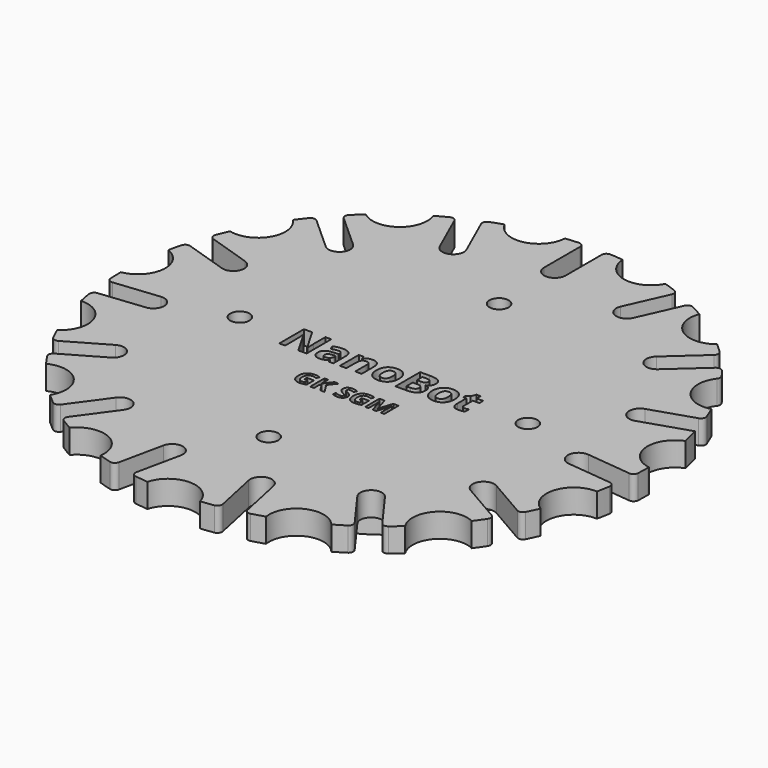
from build123d import *

# Parameters (mm, degrees)
F1_DEPTH       = 6
F2_DEPTH       = 6
F2_DEPTH_BACK  = 13
F3_DEPTH       = 2
F4_R           = 2
F5_DEPTH       = 10
F6_DEPTH       = 3
F7_TEXT_SIZE   = 8.9862398203
F7_TEXT_SIZE_2 = 5.2074857608
F8_DEPTH       = 3
F9_R           = 1
F10_DEPTH      = 1


# Not quite as in the source:
# - Text() gives the source's letters only with a copy of the font that has no kerning and outlines rounded to 1/6400 em; it was checked with that copy


with BuildPart() as f1:
    # F0 (on Top) → F1 (new body)
    with BuildSketch(Plane.XY):
        with BuildLine():
            ThreePointArc((54.8881035117, -3.5065785158), (54.9720187602, -1.7541816975), (55, 0))
            ThreePointArc((55, 0), (54.9998451105, 0.1305289846), (54.9993804431, 0.261057234))
            ThreePointArc((54.9993804431, 0.261057234), (50.2561749386, 5.2821368343), (53.8517888732, 11.1796616747))
            ThreePointArc((53.8517888732, 11.1796616747), (53.4370798147, 13.0183908712), (52.9596080906, 14.8418297689))
            Line((52.9596080906, 14.8418297689), (43.0553454731, 11.6237397678))
            ThreePointArc((43.0553454731, 11.6237397678), (40.2201800741, 13.0683286921), (41.6647689984, 15.9034940911))
            Line((41.6647689984, 15.9034940911), (51.5690316159, 19.1215840922))
            ThreePointArc((51.5690316159, 19.1215840922), (50.8835238625, 20.8774279865), (50.1382526339, 22.608751023))
            ThreePointArc((50.1382526339, 22.608751023), (43.7628617294, 25.2665), (44.6488790507, 32.1166249708))
            ThreePointArc((44.6488790507, 32.1166249708), (43.5221449332, 33.6277103058), (42.3442933924, 35.0992993819))
            Line((42.3442933924, 35.0992993819), (34.6052143911, 28.1310013499))
            ThreePointArc((34.6052143911, 28.1310013499), (31.4275946694, 28.2975333429), (31.5941266625, 31.4751530645))
            Line((31.5941266625, 31.4751530645), (39.3332056638, 38.4434510965))
            ThreePointArc((39.3332056638, 38.4434510965), (37.9927971182, 39.768673188), (36.6077654526, 41.047186366))
            ThreePointArc((36.6077654526, 41.047186366), (29.7025521541, 40.8820557767), (27.725772418, 47.5003320391))
            ThreePointArc((27.725772418, 47.5003320391), (26.0818358065, 48.4224931304), (24.4072656808, 49.2877812646))
            Line((24.4072656808, 49.2877812646), (20.1715273623, 39.7741572365))
            ThreePointArc((20.1715273623, 39.7741572365), (18.9223779691, 38.5887587238), (17.2008926357, 38.6338374037))
            Line((17.2008926357, 38.6338374037), (8.7448378261, 19.6412273393))
            ThreePointArc((8.7448378261, 19.6412273393), (18.0314172108, 11.7097392528), (21.5, 0))
            ThreePointArc((21.5, 0), (16.8782404296, -13.3182206019), (5, -20.9105236663))
            ThreePointArc((5, -20.9105236663), (0, -21.5), (-5, -20.9105236663))
            ThreePointArc((-5, -20.9105236663), (-21.3521223632, 2.5173141614), (0, 21.5))
            Line((0, 21.5), (0, 42.29))
            ThreePointArc((0, 42.29), (-1.5909902577, 42.9490097423), (-2.25, 44.54))
            Line((-2.25, 44.54), (-2.25, 54.9539580012))
            ThreePointArc((-2.25, 54.9539580012), (-4.1317403228, 54.8445869882), (-6.0086278536, 54.6708001708))
            ThreePointArc((-6.0086278536, 54.6708001708), (-10.5064014721, 49.4287327079), (-16.7474630535, 52.3881902844))
            ThreePointArc((-16.7474630535, 52.3881902844), (-18.5327705984, 51.7835535083), (-20.2963111214, 51.1180961584))
            Line((-20.2963111214, 51.1180961584), (-16.0605728029, 41.6044721303))
            ThreePointArc((-16.0605728029, 41.6044721303), (-17.2008926357, 38.6338374037), (-20.1715273623, 39.7741572365))
            Line((-20.1715273623, 39.7741572365), (-24.4072656808, 49.2877812646))
            ThreePointArc((-24.4072656808, 49.2877812646), (-26.0818358065, 48.4224931304), (-27.725772418, 47.5003320391))
            ThreePointArc((-27.725772418, 47.5003320391), (-27.4499898145, 46.5095766113), (-27.3570502396, 45.4853624747))
            ThreePointArc((-27.3570502396, 45.4853624747), (-30.5857873079, 40.3552275076), (-36.6077654526, 41.047186366))
            ThreePointArc((-36.6077654526, 41.047186366), (-37.9927971182, 39.768673188), (-39.3332056638, 38.4434510965))
            Line((-39.3332056638, 38.4434510965), (-31.5941266625, 31.4751530645))
            ThreePointArc((-31.5941266625, 31.4751530645), (-31.4275946694, 28.2975333429), (-34.6052143911, 28.1310013499))
            Line((-34.6052143911, 28.1310013499), (-42.3442933924, 35.0992993819))
            ThreePointArc((-42.3442933924, 35.0992993819), (-43.5221449332, 33.6277103058), (-44.6488790507, 32.1166249708))
            ThreePointArc((-44.6488790507, 32.1166249708), (-43.4287411439, 30.2770268969), (-43.000546277, 28.1115))
            ThreePointArc((-43.000546277, 28.1115), (-45.2164528104, 23.6051961281), (-50.1382526339, 22.608751023))
            ThreePointArc((-50.1382526339, 22.608751023), (-50.8835238625, 20.8774279865), (-51.5690316159, 19.1215840922))
            Line((-51.5690316159, 19.1215840922), (-41.6647689984, 15.9034940911))
            ThreePointArc((-41.6647689984, 15.9034940911), (-40.2201800741, 13.0683286921), (-43.0553454731, 11.6237397678))
            Line((-43.0553454731, 11.6237397678), (-52.9596080906, 14.8418297689))
            ThreePointArc((-52.9596080906, 14.8418297689), (-53.4370798147, 13.0183908712), (-53.8517888732, 11.1796616747))
            ThreePointArc((-53.8517888732, 11.1796616747), (-51.2184208155, 9.0890995308), (-50.2250045233, 5.8769037903))
            ThreePointArc((-50.2250045233, 5.8769037903), (-51.5799150769, 2.1913781166), (-54.9993804431, 0.261057234))
            ThreePointArc((-54.9993804431, 0.261057234), (-54.9760270687, -1.6237141794), (-54.8881035117, -3.5065785158))
            Line((-54.8881035117, -3.5065785158), (-44.5311942621, -2.4180234894))
            ThreePointArc((-44.5311942621, -2.4180234894), (-42.0583309551, -4.4205087116), (-44.0608161774, -6.8933720185))
            Line((-44.0608161774, -6.8933720185), (-54.417725427, -7.9819270449))
            ThreePointArc((-54.417725427, -7.9819270449), (-54.1122581356, -9.8419266134), (-53.7432351713, -11.690366689))
            ThreePointArc((-53.7432351713, -11.690366689), (-49.5451514779, -13.2553862583), (-47.7812505157, -17.3738624747))
            ThreePointArc((-47.7812505157, -17.3738624747), (-48.4646293003, -20.0775347933), (-50.3506157199, -22.1317757223))
            ThreePointArc((-50.3506157199, -22.1317757223), (-49.5626757532, -23.8441014127), (-48.7165236676, -25.5284218421))
            Line((-48.7165236676, -25.5284218421), (-39.6977714846, -20.3214428415))
            ThreePointArc((-39.6977714846, -20.3214428415), (-36.624214326, -21.145), (-37.4477714846, -24.2185571585))
            Line((-37.4477714846, -24.2185571585), (-46.4665236676, -29.4255361591))
            ThreePointArc((-46.4665236676, -29.4255361591), (-45.4309354304, -31.0004855755), (-44.3419878664, -32.5390244485))
            ThreePointArc((-44.3419878664, -32.5390244485), (-38.7978065225, -32.7757705623), (-36.0918315228, -37.6205300813))
            ThreePointArc((-36.0918315228, -37.6205300813), (-36.3224919101, -39.2241855907), (-36.9957721178, -40.6978235954))
            ThreePointArc((-36.9957721178, -40.6978235954), (-35.5794875372, -41.9416268949), (-34.1214143056, -43.1361691135))
            Line((-34.1214143056, -43.1361691135), (-28.0002433745, -34.7111001118))
            ThreePointArc((-28.0002433745, -34.7111001118), (-24.8574383194, -34.2133286921), (-24.3596668998, -37.3561337471))
            Line((-24.3596668998, -37.3561337471), (-30.4808378309, -45.7812027488))
            ThreePointArc((-30.4808378309, -45.7812027488), (-28.8941912622, -46.798778951), (-27.273608025, -47.7613892731))
            ThreePointArc((-27.273608025, -47.7613892731), (-20.9564195323, -46.0029626821), (-17.1779542837, -51.362266265))
            ThreePointArc((-17.1779542837, -51.362266265), (-17.1944956114, -51.7958175243), (-17.2440234205, -52.2268480408))
            ThreePointArc((-17.2440234205, -52.2268480408), (-15.4442826965, -52.7870640592), (-13.6264024268, -53.2852808654))
            Line((-13.6264024268, -53.2852808654), (-11.4612188107, -43.0988928323))
            ThreePointArc((-11.4612188107, -43.0988928323), (-8.7925854047, -41.365862035), (-7.0595546074, -44.034495441))
            Line((-7.0595546074, -44.034495441), (-9.2247382235, -54.2208834741))
            ThreePointArc((-9.2247382235, -54.2208834741), (-7.3613789293, -54.5051382923), (-5.4893735832, -54.7253759938))
            ThreePointArc((-5.4893735832, -54.7253759938), (0, -50.533), (5.4893735832, -54.7253759938))
            ThreePointArc((5.4893735832, -54.7253759938), (7.3613789293, -54.5051382923), (9.2247382235, -54.2208834741))
            Line((9.2247382235, -54.2208834741), (7.0595546074, -44.034495441))
            ThreePointArc((7.0595546074, -44.034495441), (8.7925854047, -41.365862035), (11.4612188107, -43.0988928323))
            Line((11.4612188107, -43.0988928323), (13.6264024268, -53.2852808654))
            ThreePointArc((13.6264024268, -53.2852808654), (15.4442826965, -52.7870640592), (17.2440234205, -52.2268480408))
            ThreePointArc((17.2440234205, -52.2268480408), (20.5536227845, -46.1641926111), (27.273608025, -47.7613892731))
            ThreePointArc((27.273608025, -47.7613892731), (28.8941912622, -46.798778951), (30.4808378309, -45.7812027488))
            Line((30.4808378309, -45.7812027488), (24.3596668998, -37.3561337471))
            ThreePointArc((24.3596668998, -37.3561337471), (24.8574383194, -34.2133286921), (28.0002433745, -34.7111001118))
            Line((28.0002433745, -34.7111001118), (34.1214143056, -43.1361691135))
            ThreePointArc((34.1214143056, -43.1361691135), (35.5794875372, -41.9416268949), (36.9957721178, -40.6978235954))
            ThreePointArc((36.9957721178, -40.6978235954), (37.5533374658, -33.8131769311), (44.3419878664, -32.5390244485))
            ThreePointArc((44.3419878664, -32.5390244485), (45.4309354304, -31.0004855755), (46.4665236676, -29.4255361591))
            Line((46.4665236676, -29.4255361591), (37.4477714846, -24.2185571585))
            ThreePointArc((37.4477714846, -24.2185571585), (36.624214326, -21.145), (39.6977714846, -20.3214428415))
            Line((39.6977714846, -20.3214428415), (48.7165236676, -25.5284218421))
            ThreePointArc((48.7165236676, -25.5284218421), (49.5626757532, -23.8441014127), (50.3506157199, -22.1317757223))
            ThreePointArc((50.3506157199, -22.1317757223), (48.0597389379, -15.6155557767), (53.7432351713, -11.690366689))
            ThreePointArc((53.7432351713, -11.690366689), (54.1122581356, -9.8419266134), (54.417725427, -7.9819270449))
            Line((54.417725427, -7.9819270449), (44.0608161774, -6.8933720185))
            ThreePointArc((44.0608161774, -6.8933720185), (42.0583309551, -4.4205087116), (44.5311942621, -2.4180234894))
            Line((44.5311942621, -2.4180234894), (54.8881035117, -3.5065785158))
        make_face()
        with BuildLine():
            Line((4.4701013526, 21.0301734158), (10.5064014721, 49.4287327079))
            ThreePointArc((10.5064014721, 49.4287327079), (7.3711108575, 51.2892184916), (6.0086278536, 54.6708001708))
            ThreePointArc((6.0086278536, 54.6708001708), (4.1317403228, 54.8445869882), (2.25, 54.9539580012))
            Line((2.25, 54.9539580012), (2.25, 44.54))
            ThreePointArc((2.25, 44.54), (1.5909902577, 42.9490097423), (0, 42.29))
            Line((0, 42.29), (0, 21.5))
            ThreePointArc((0, 21.5), (2.2473619603, 21.3822207504), (4.4701013526, 21.0301734158))
        make_face()
        with BuildLine():
            Line((16.0605728029, 41.6044721303), (20.2963111214, 51.1180961584))
            ThreePointArc((20.2963111214, 51.1180961584), (18.5327705984, 51.7835535083), (16.7474630535, 52.3881902844))
            ThreePointArc((16.7474630535, 52.3881902844), (14.1273597136, 49.8531334649), (10.5064014721, 49.4287327079))
            Line((10.5064014721, 49.4287327079), (4.4701013526, 21.0301734158))
            ThreePointArc((4.4701013526, 21.0301734158), (6.6438653791, 20.4477151003), (8.7448378261, 19.6412273393))
            Line((8.7448378261, 19.6412273393), (17.2008926357, 38.6338374037))
            ThreePointArc((17.2008926357, 38.6338374037), (16.015494123, 39.8829867969), (16.0605728029, 41.6044721303))
        make_face()
    extrude(amount=F1_DEPTH)



with BuildPart() as f1b:
    # F0 (on Top) → F1, piece 2 (new body)
    with BuildSketch(Plane.XY):
        with BuildLine():
            ThreePointArc((17.5, 0), (14.676734939, 9.5311831128), (7.1178912538, 15.9870455087))
            Line((7.1178912538, 15.9870455087), (5.0842080384, 11.4193182205))
            ThreePointArc((5.0842080384, 11.4193182205), (10.4833820993, 6.8079879377), (12.5, 0))
            ThreePointArc((12.5, 0), (-8.8388347648, -8.8388347648), (0, 12.5))
            Line((0, 12.5), (0, 17.5))
            ThreePointArc((0, 17.5), (-12.3743686708, -12.3743686708), (17.5, 0))
        make_face()
        with BuildLine():
            Line((5.0842080384, 11.4193182205), (7.1178912538, 15.9870455087))
            ThreePointArc((7.1178912538, 15.9870455087), (5.4077974016, 16.6434890352), (3.6384545893, 17.1175830128))
            Line((3.6384545893, 17.1175830128), (2.5988961352, 12.2268450092))
            ThreePointArc((2.5988961352, 12.2268450092), (3.8627124297, 11.8882064537), (5.0842080384, 11.4193182205))
        make_face()
        with BuildLine():
            Line((2.5988961352, 12.2268450092), (3.6384545893, 17.1175830128))
            ThreePointArc((3.6384545893, 17.1175830128), (1.8292481072, 17.4041331689), (0, 17.5))
            Line((0, 17.5), (0, 12.5))
            ThreePointArc((0, 12.5), (1.3066057908, 12.4315236921), (2.5988961352, 12.2268450092))
        make_face()
        with BuildLine():
            ThreePointArc((12.5, 0), (10.4833820993, 6.8079879377), (5.0842080384, 11.4193182205))
            Line((5.0842080384, 11.4193182205), (0, 0))
            Line((0, 0), (0, 12.5))
            ThreePointArc((0, 12.5), (-8.8388347648, -8.8388347648), (12.5, 0))
        make_face()
        with BuildLine():
            Line((0, 0), (5.0842080384, 11.4193182205))
            ThreePointArc((5.0842080384, 11.4193182205), (3.8627124297, 11.8882064537), (2.5988961352, 12.2268450092))
            Line((2.5988961352, 12.2268450092), (0, 0))
        make_face()
        with BuildLine():
            Line((0, 12.5), (0, 0))
            Line((0, 0), (2.5988961352, 12.2268450092))
            ThreePointArc((2.5988961352, 12.2268450092), (1.3066057908, 12.4315236921), (0, 12.5))
        make_face()
    extrude(amount=F1_DEPTH)


with BuildPart() as f1_1:
    add(f1.part)

    add(f1b.part)  # F2 merges F1b
    # F0 (on Top) → F2 (join, two sides)
    with BuildSketch(Plane.XY) as f2_sk:
        with BuildLine():
            ThreePointArc((21.5, 0), (18.0314172108, 11.7097392528), (8.7448378261, 19.6412273393))
            Line((8.7448378261, 19.6412273393), (7.1178912538, 15.9870455087))
            ThreePointArc((7.1178912538, 15.9870455087), (14.676734939, 9.5311831128), (17.5, 0))
            ThreePointArc((17.5, 0), (-12.3743686708, -12.3743686708), (0, 17.5))
            Line((0, 17.5), (0, 21.5))
            ThreePointArc((0, 21.5), (-21.3521223632, 2.5173141614), (-5, -20.9105236663))
            ThreePointArc((-5, -20.9105236663), (0, -21.5), (5, -20.9105236663))
            ThreePointArc((5, -20.9105236663), (16.8782404296, -13.3182206019), (21.5, 0))
        make_face()
        with BuildLine():
            Line((7.1178912538, 15.9870455087), (8.7448378261, 19.6412273393))
            ThreePointArc((8.7448378261, 19.6412273393), (6.6438653791, 20.4477151003), (4.4701013526, 21.0301734158))
            Line((4.4701013526, 21.0301734158), (3.6384545893, 17.1175830128))
            ThreePointArc((3.6384545893, 17.1175830128), (5.4077974016, 16.6434890352), (7.1178912538, 15.9870455087))
        make_face()
        with BuildLine():
            Line((3.6384545893, 17.1175830128), (4.4701013526, 21.0301734158))
            ThreePointArc((4.4701013526, 21.0301734158), (2.2473619603, 21.3822207504), (0, 21.5))
            Line((0, 21.5), (0, 17.5))
            ThreePointArc((0, 17.5), (1.8292481072, 17.4041331689), (3.6384545893, 17.1175830128))
        make_face()
    extrude(amount=F2_DEPTH)
    extrude(f2_sk.sketch, amount=-F2_DEPTH_BACK)

    # F0 (on Top) → F3 (join)
    with BuildSketch(Plane.XY):
        with BuildLine():
            Line((2.5988961352, 12.2268450092), (3.6384545893, 17.1175830128))
            ThreePointArc((3.6384545893, 17.1175830128), (1.8292481072, 17.4041331689), (0, 17.5))
            Line((0, 17.5), (0, 12.5))
            ThreePointArc((0, 12.5), (1.3066057908, 12.4315236921), (2.5988961352, 12.2268450092))
        make_face()
        with BuildLine():
            Line((5.0842080384, 11.4193182205), (7.1178912538, 15.9870455087))
            ThreePointArc((7.1178912538, 15.9870455087), (5.4077974016, 16.6434890352), (3.6384545893, 17.1175830128))
            Line((3.6384545893, 17.1175830128), (2.5988961352, 12.2268450092))
            ThreePointArc((2.5988961352, 12.2268450092), (3.8627124297, 11.8882064537), (5.0842080384, 11.4193182205))
        make_face()
        with BuildLine():
            ThreePointArc((17.5, 0), (14.676734939, 9.5311831128), (7.1178912538, 15.9870455087))
            Line((7.1178912538, 15.9870455087), (5.0842080384, 11.4193182205))
            ThreePointArc((5.0842080384, 11.4193182205), (10.4833820993, 6.8079879377), (12.5, 0))
            ThreePointArc((12.5, 0), (-8.8388347648, -8.8388347648), (0, 12.5))
            Line((0, 12.5), (0, 17.5))
            ThreePointArc((0, 17.5), (-12.3743686708, -12.3743686708), (17.5, 0))
        make_face()
    extrude(amount=-F3_DEPTH)

    # F4 (on face) → F5 (cut)
    with BuildSketch(Plane(origin=(0, 0, 0), x_dir=(1, 0, 0), z_dir=(0, 0, -1))):
        with Locations((-30, 0)):
            Circle(F4_R)
        with Locations((0, 30)):
            Circle(F4_R)
        with Locations((30, 0)):
            Circle(F4_R)
        with Locations((0, -30)):
            Circle(F4_R)
    extrude(amount=-F5_DEPTH, mode=Mode.SUBTRACT)

    # F4 (on face) → F6 (cut)
    with BuildSketch(Plane(origin=(0, 0, 0), x_dir=(1, 0, 0), z_dir=(0, 0, -1))):
        Polygon((-3, -28.2679491924), (-3, -31.7320508076), (0, -33.4641016151), (3, -31.7320508076), (3, -28.2679491924), (0, -26.5358983849), align=None)
        with Locations((0, -30)):
            Circle(F4_R, mode=Mode.SUBTRACT)
        Polygon((-26.5358983849, 0), (-28.2679491924, 3), (-31.7320508076, 3), (-33.4641016151, 0), (-31.7320508076, -3), (-28.2679491924, -3), align=None)
        with Locations((-30, 0)):
            Circle(F4_R, mode=Mode.SUBTRACT)
        Polygon((3, 28.2679491924), (3, 31.7320508076), (0, 33.4641016151), (-3, 31.7320508076), (-3, 28.2679491924), (0, 26.5358983849), align=None)
        with Locations((0, 30)):
            Circle(F4_R, mode=Mode.SUBTRACT)
        Polygon((28.2679491924, -3), (31.7320508076, -3), (33.4641016151, 0), (31.7320508076, 3), (28.2679491924, 3), (26.5358983849, 0), align=None)
        with Locations((30, 0)):
            Circle(F4_R, mode=Mode.SUBTRACT)
    extrude(amount=-F6_DEPTH, mode=Mode.SUBTRACT)

    # F7 (on face) → F8 (cut)
    with BuildSketch(Plane.XY.offset(6)):
        with Locations((-20, -3.2350926706)):
            Text('NanoBot', F7_TEXT_SIZE, font='Open Sans', font_style=FontStyle.BOLD, text_align=(TextAlign.LEFT, TextAlign.BOTTOM))
        with Locations((-10, -11.9844824184)):
            Text('GK SGM', F7_TEXT_SIZE_2, font='Open Sans', font_style=FontStyle.BOLD, text_align=(TextAlign.LEFT, TextAlign.BOTTOM))
    extrude(amount=-F8_DEPTH, mode=Mode.SUBTRACT)

    # F9
    f9_edges = [f1_1.edges().sort_by_distance(p)[0] for p in [
        (48.716524, -25.528422, 3),
        (46.466524, -29.425536, 3),
        (34.121414, -43.136169, 3),
        (30.480838, -45.781203, 3),
        (13.626402, -53.285281, 3),
        (9.224738, -54.220883, 3),
        (-9.224738, -54.220883, 3),
        (54.417725, -7.981927, 3),
        (54.888104, -3.506579, 3),
        (51.569032, 19.121584, 3),
        (44.648879, 32.116625, 3),
        (-13.626402, -53.285281, 3),
        (-30.480838, -45.781203, 3),
        (-34.121414, -43.136169, 3),
        (-46.466524, -29.425536, 3),
        (-48.716524, -25.528422, 3),
        (-54.417725, -7.981927, 3),
        (-54.888104, -3.506579, 3),
        (-52.959608, 14.84183, 3),
        (-51.569032, 19.121584, 3),
        (-42.344293, 35.099299, 3),
        (-39.333206, 38.443451, 3),
        (-24.407266, 49.287781, 3),
        (-20.296311, 51.118096, 3),
        (2.25, 54.953958, 3),
        (-2.25, 54.953958, 3),
        (20.296311, 51.118096, 3),
        (24.407266, 49.287781, 3),
        (39.333206, 38.443451, 3),
        (42.344293, 35.099299, 3),
    ]]
    fillet(f9_edges, radius=F9_R)

    # F10 (cut): a face of the model
    f10_faces = [f1_1.faces().sort_by_distance(p)[0] for p in [
        (48.5538950154, -8.9271710949, 0),
    ]]
    extrude(f10_faces, amount=-F10_DEPTH, mode=Mode.SUBTRACT)


solid = f1_1.part
